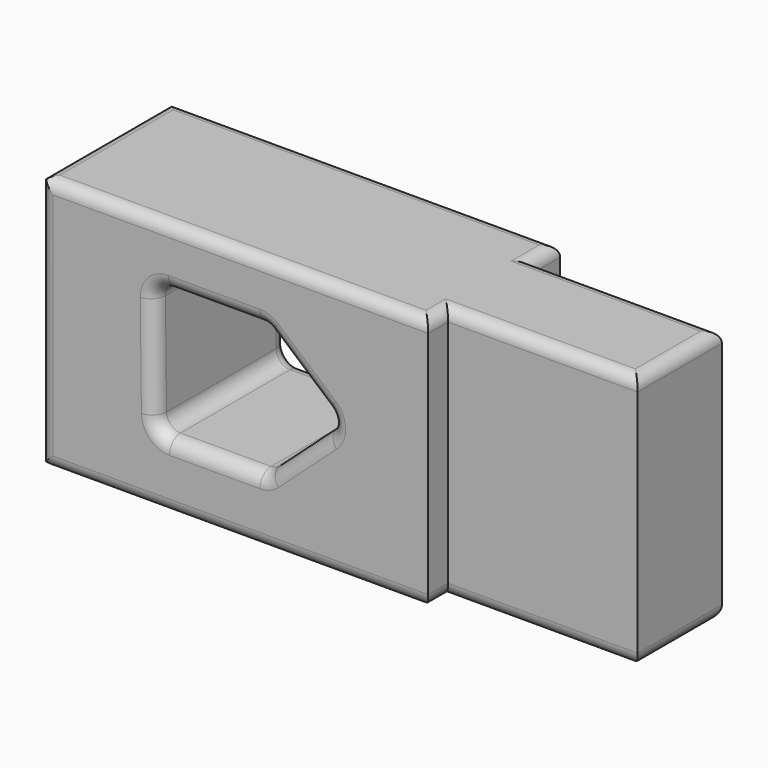
from build123d import *

# Parameters (mm, degrees)
F0_W        = 68.9248368144
F0_H        = 38.2718367036
F1_DEPTH    = 92.964
F2_R        = 4.2924717139
F3_R        = 5.08
F4_T1_DEPTH = 108.9915282861
F6_DEPTH    = 66.294
F7_R        = 5.08


# Not quite as in the source:
# - a fillet or chamfer that OpenCascade refuses, or shapes differently, is made with other operations: its cross-section is extruded or revolved along the edge and cut away or added


with BuildPart() as f1:
    # F0 (on Top) → F1 (new body)
    with BuildSketch(Plane.XY):
        Polygon((-76.8856033683, 47.9822456837), (-76.8856033683, -11.9746578857), (64.6745637059, -11.9746578857), (64.6745637059, -2.9509027954), (64.6745637059, 35.3209339082), (64.6745637059, 47.9822456837), align=None)
        with Locations((99.1369821131, 16.1850155564)):
            Rectangle(F0_W, F0_H)
    extrude(amount=F1_DEPTH)

    # F2
    f2_edges = [f1.edges().sort_by_distance(p)[0] for p in [
        (-76.885603, 18.003794, 92.964),
        (-6.10552, -11.974658, 92.964),
        (64.674564, -7.46278, 92.964),
        (99.136982, -2.950903, 92.964),
        (133.599401, 16.185016, 92.964),
        (99.136982, 35.320934, 92.964),
        (64.674564, 41.65159, 92.964),
        (-6.10552, 47.982246, 92.964),
    ]]
    fillet(f2_edges, radius=F2_R)

    # F3
    f3_edges = [f1.edges().sort_by_distance(p)[0] for p in [
        (99.136982, -2.950903, 0),
        (-76.885603, 18.003794, 0),
        (-6.10552, -11.974658, 0),
        (64.674564, -7.46278, 0),
        (133.599401, 16.185016, 0),
        (99.136982, 35.320934, 0),
        (64.674564, 41.65159, 0),
        (-6.10552, 47.982246, 0),
    ]]
    fillet(f3_edges, radius=F3_R)

    # F4: fillet of radius 5.08 on 4 edges, made by hand

    # F4_s2 → F4_t1 (cut)
    with BuildSketch(Plane.XY.offset(-7.62)):
        with BuildLine():
            ThreePointArc((-76.8856033683, 42.9022456837), (-75.3977058167, 46.4943481321), (-71.8056033683, 47.9822456837))
            Line((-71.8056033683, 47.9822456837), (-76.8856033683, 47.9822456837))
            Line((-76.8856033683, 47.9822456837), (-76.8856033683, 42.9022456837))
        make_face()
        with BuildLine():
            ThreePointArc((-76.8856033683, -6.8946578857), (-75.3977058167, -10.4867603342), (-71.8056033683, -11.9746578857))
            Line((-71.8056033683, -11.9746578857), (-76.8856033683, -11.9746578857))
            Line((-76.8856033683, -11.9746578857), (-76.8856033683, -6.8946578857))
        make_face()
    extrude(amount=F4_T1_DEPTH, mode=Mode.SUBTRACT)

    # F5 (on face) → F6 (cut)
    with BuildSketch(Plane(origin=(0, 47.9822456837, 0), x_dir=(-1, 0, 0), z_dir=(0, 1, 0))):
        Polygon((34.4493128359, 24.1737514734), (34.9953584373, 71.4389234781), (-5.412035156, 71.4389234781), (-32.1682840586, 48.3612157404), (-5.412035156, 24.1737514734), align=None)
    extrude(amount=-F6_DEPTH, mode=Mode.SUBTRACT)

    # F7
    f7_edges = [f1.edges().sort_by_distance(p)[0] for p in [
        (-34.722336, 47.982246, 47.806337),
        (-34.995358, 18.003794, 71.438923),
        (-34.722336, -11.974658, 47.806337),
        (-34.449313, 18.003794, 24.173751),
        (18.79016, 47.982246, 59.90007),
        (32.168284, 18.003794, 48.361216),
        (18.79016, -11.974658, 59.90007),
        (5.412035, 18.003794, 71.438923),
        (18.79016, 47.982246, 36.267484),
        (5.412035, 18.003794, 24.173751),
        (18.79016, -11.974658, 36.267484),
        (-14.791662, -11.974658, 71.438923),
        (-14.518639, -11.974658, 24.173751),
        (-14.518639, 47.982246, 24.173751),
        (-14.791662, 47.982246, 71.438923),
    ]]
    fillet(f7_edges, radius=F7_R)


solid = f1.part
